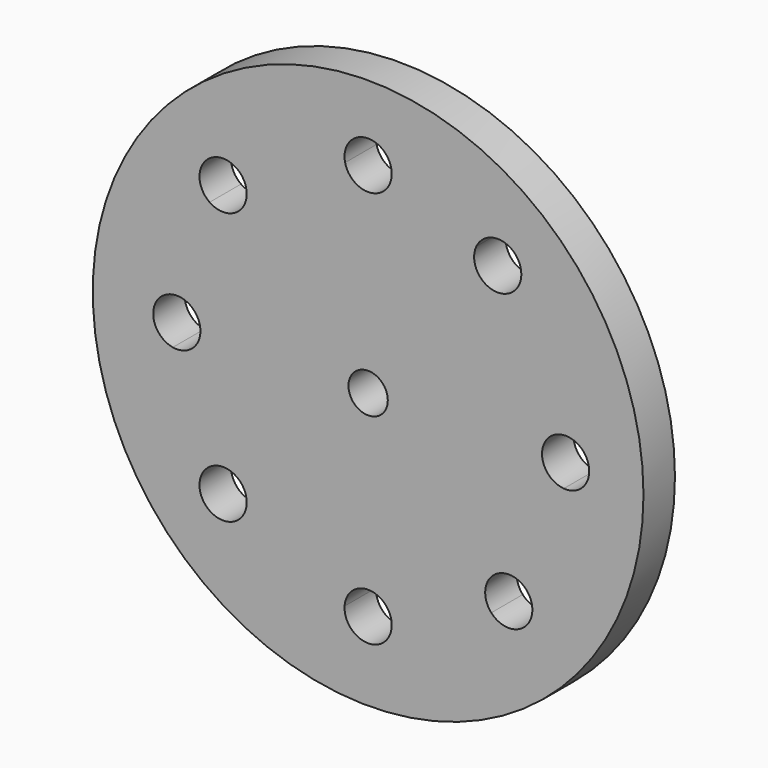
from build123d import *

# Parameters (mm, degrees)
F0_R     = 17.5
F0_R_2   = 2.5
F0_R_3   = 1.25
F1_DEPTH = 2.5


# Not quite as in the source:
# - the program builds the solid bodies; features that only make, move or delete a surface that nothing else refers to are left out


with BuildPart() as f1:
    # F0 (on Front) → F1 (new body)
    with BuildSketch(Plane.XZ):
        Circle(F0_R)
        with BuildLine():
            ThreePointArc((1.4972975656, -12.41), (1.4993242392, -12.454979718), (1.5, -12.5))
            ThreePointArc((1.5, -12.5), (-0.045020282, -13.9993242392), (-1.4972975656, -12.41))
            ThreePointArc((-1.4972975656, -12.41), (-4.9790100681, -11.4655771221), (-8.0460146394, -9.5661720883))
            ThreePointArc((-8.0460146394, -9.5661720883), (-10.3118696418, -9.6536659725), (-10.0753310722, -7.3984933456))
            ThreePointArc((-10.0753310722, -7.3984933456), (-11.6269109472, -4.5896559594), (-12.4122705024, -1.4783575263))
            ThreePointArc((-12.4122705024, -1.4783575263), (-13.658382684, 0), (-12.4122705024, 1.4783575263))
            ThreePointArc((-12.4122705024, 1.4783575263), (-11.6269110451, 4.5896557115), (-10.0753313878, 7.3984929159))
            ThreePointArc((-10.0753313878, 7.3984929159), (-10.3118706248, 9.6536659173), (-8.0460151958, 9.5661716203))
            ThreePointArc((-8.0460151958, 9.5661716203), (-4.9630114991, 11.472511358), (-1.4626687852, 12.4141290482))
            ThreePointArc((-1.4626687852, 12.4141290482), (-0.167324239, 14.2373289873), (1.5000009313, 12.7466907725))
            ThreePointArc((1.5000009313, 12.7466907725), (1.4906391339, 12.5793654932), (1.4626705992, 12.4141288344))
            ThreePointArc((1.4626705992, 12.4141288344), (4.2850452641, 11.7425886024), (6.8765961266, 10.4385068718))
            ThreePointArc((6.8765961266, 10.4385068718), (8.5606760335, 11.2696593384), (9.736322552, 9.8051475361))
            ThreePointArc((9.736322552, 9.8051475361), (9.5663280132, 9.1115442827), (9.0948752545, 8.5751527162))
            ThreePointArc((9.0948752545, 8.5751527162), (11.2789515194, 5.388436937), (12.3856373166, 1.6870057091))
            ThreePointArc((12.3856373166, 1.6870057091), (13.5512317227, 1.3135614646), (14.0505886972, 0.1961029484))
            ThreePointArc((14.0505886972, 0.1961029484), (13.5685677546, -0.9055860452), (12.4322971789, -1.2992254827))
            ThreePointArc((12.4322971789, -1.2992254827), (11.6124376907, -4.6261529244), (9.9200203194, -7.6054715083))
            ThreePointArc((9.9200203194, -7.6054715083), (10.3020717987, -8.1159348628), (10.4375838551, -8.7389698954))
            ThreePointArc((10.4375838551, -8.7389698954), (9.4776271369, -10.1383816482), (7.8264461833, -9.7466271161))
            ThreePointArc((7.8264461833, -9.7466271161), (4.8483438568, -11.5214392263), (1.4972975656, -12.41))
        make_face(mode=Mode.SUBTRACT)
        with BuildLine():
            ThreePointArc((-1.4972975656, -12.41), (0, -11), (1.4972975656, -12.41))
            ThreePointArc((1.4972975656, -12.41), (4.8483438568, -11.5214392263), (7.8264461833, -9.7466271161))
            ThreePointArc((7.8264461833, -9.7466271161), (7.8650737925, -7.690293508), (9.9200203194, -7.6054715083))
            ThreePointArc((9.9200203194, -7.6054715083), (11.6124376907, -4.6261529244), (12.4322971789, -1.2992254827))
            ThreePointArc((12.4322971789, -1.2992254827), (11.0507717691, 0.1726683089), (12.3856373166, 1.6870057091))
            ThreePointArc((12.3856373166, 1.6870057091), (11.2789515194, 5.388436937), (9.0948752545, 8.5751527162))
            ThreePointArc((9.0948752545, 8.5751527162), (7.271534517, 8.6565901594), (6.8765961266, 10.4385068718))
            ThreePointArc((6.8765961266, 10.4385068718), (4.2850452641, 11.7425886024), (1.4626705992, 12.4141288344))
            ThreePointArc((1.4626705992, 12.4141288344), (8.217e-07, 11.2466907725), (-1.4626687852, 12.4141290482))
            ThreePointArc((-1.4626687852, 12.4141290482), (-4.9630114991, 11.472511358), (-8.0460151958, 9.5661716203))
            ThreePointArc((-8.0460151958, 9.5661716203), (-7.8015231838, 9.1254022263), (-7.7168385163, 8.6285294965))
            ThreePointArc((-7.7168385163, 8.6285294965), (-8.5232029157, 7.298540905), (-10.0753313878, 7.3984929159))
            ThreePointArc((-10.0753313878, 7.3984929159), (-11.6269110451, 4.5896557115), (-12.4122705024, 1.4783575263))
            ThreePointArc((-12.4122705024, 1.4783575263), (-11.1916437657, 1.146915805), (-10.658382684, 0))
            ThreePointArc((-10.658382684, 0), (-11.1916437657, -1.146915805), (-12.4122705024, -1.4783575263))
            ThreePointArc((-12.4122705024, -1.4783575263), (-11.6269109472, -4.5896559594), (-10.0753310722, -7.3984933456))
            ThreePointArc((-10.0753310722, -7.3984933456), (-8.5232023173, -7.2985407313), (-7.716837585, -8.6285294965))
            ThreePointArc((-7.716837585, -8.6285294965), (-7.8015223518, -9.1254025092), (-8.0460146394, -9.5661720883))
            ThreePointArc((-8.0460146394, -9.5661720883), (-4.9790100681, -11.4655771221), (-1.4972975656, -12.41))
        make_face()
        Circle(F0_R_2, mode=Mode.SUBTRACT)
        Circle(F0_R_2)
        Circle(F0_R_3, mode=Mode.SUBTRACT)
    extrude(amount=F1_DEPTH)


solid = f1.part
